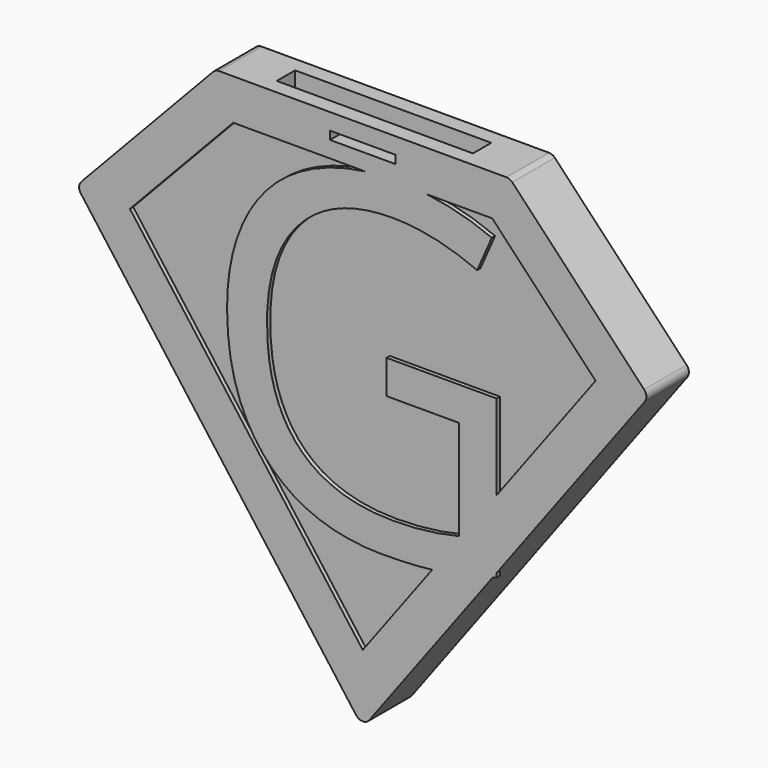
from build123d import *

# Parameters (mm, degrees)
F1_DEPTH     = 3.25
F3_DEPTH     = 0.5
F5_DEPTH     = 0.5
F6_TEXT_SIZE = 55.5555555556
F7_DEPTH     = 0.5
F8_TEXT_SIZE = 55.5555555556
F9_DEPTH     = 0.5
F10_W        = 24
F10_H        = 2.8
F11_DEPTH    = 20
F13_DEPTH    = 1.4
F14_W        = 8
F14_H        = 1
F15_DEPTH    = 25
F16_R        = 1


# Not quite as in the source:
# - Text() gives the source's letters only with a copy of the font that has no kerning and outlines rounded to 1/6400 em; it was checked with that copy


with BuildPart() as f1:
    # F0 (on Front) → F1 (new body, symmetric)
    with BuildSketch(Plane.XZ):
        Polygon((18, 18), (0, 18), (-18, 18), (-35, 0), (0, -47), (35, 0), align=None)
    extrude(amount=F1_DEPTH, both=True)

    # F2 (on face) → F3 (cut)
    with BuildSketch(Plane.XZ.offset(3.25)):
        Polygon((15.8447675538, 13), (-15.8447675538, 13), (-28.4822773709, -0.3808927475), (1.162e-07, -38.628522516), (28.4822775009, -0.3808928851), align=None)
    extrude(amount=-F3_DEPTH, mode=Mode.SUBTRACT)

    # F4 (on face) → F5 (cut)
    with BuildSketch(Plane(origin=(0, 3.25, 0), x_dir=(-1, 0, 0), z_dir=(0, 1, 0))):
        Polygon((28.482277527, -0.3808925379), (15.8447676545, 13.0000002682), (-15.8447670441, 13.0000002682), (-28.4822772579, -0.3808928993), (0, -38.6285223599), align=None)
    extrude(amount=-F5_DEPTH, mode=Mode.SUBTRACT)

    # F6 (on face) → F7 (join)
    with BuildSketch(Plane.XZ.offset(2.75)):
        with Locations((-19.9913194444, -27)):
            Text('G', F6_TEXT_SIZE, font='Open Sans', text_align=(TextAlign.LEFT, TextAlign.BOTTOM))
    extrude(amount=F7_DEPTH)

    # F8 (on face) → F9 (join)
    with BuildSketch(Plane(origin=(0, 2.75, 0), x_dir=(-1, 0, 0), z_dir=(0, 1, 0))):
        with Locations((-19.9913194444, -26.9999997318)):
            Text('G', F8_TEXT_SIZE, font='Open Sans', text_align=(TextAlign.LEFT, TextAlign.BOTTOM))
    extrude(amount=F9_DEPTH)

    # F10 (on face) → F11 (cut)
    with BuildSketch(Plane.XY.offset(18)):
        Rectangle(F10_W, F10_H)
    extrude(amount=-F11_DEPTH, mode=Mode.SUBTRACT)

    # F12 (on Front) → F13 (cut, symmetric)
    with BuildSketch(Plane.XZ):
        with BuildLine():
            Line((12, -2), (-12, -2))
            ThreePointArc((-12, -2), (0, -14), (12, -2))
        make_face()
    extrude(amount=F13_DEPTH, both=True, mode=Mode.SUBTRACT)

    # F14 (on face) → F15 (cut)
    with BuildSketch(Plane.XZ.offset(3.25)):
        with Locations((0, 15.5)):
            Rectangle(F14_W, F14_H)
    extrude(amount=-F15_DEPTH, mode=Mode.SUBTRACT)

    # F16
    f16_edges = [f1.edges().sort_by_distance(p)[0] for p in [
        (0, 0, -47),
        (35, 0, 0),
        (-35, 0, 0),
        (-18, 0, 18),
        (18, 0, 18),
    ]]
    fillet(f16_edges, radius=F16_R)


solid = f1.part
